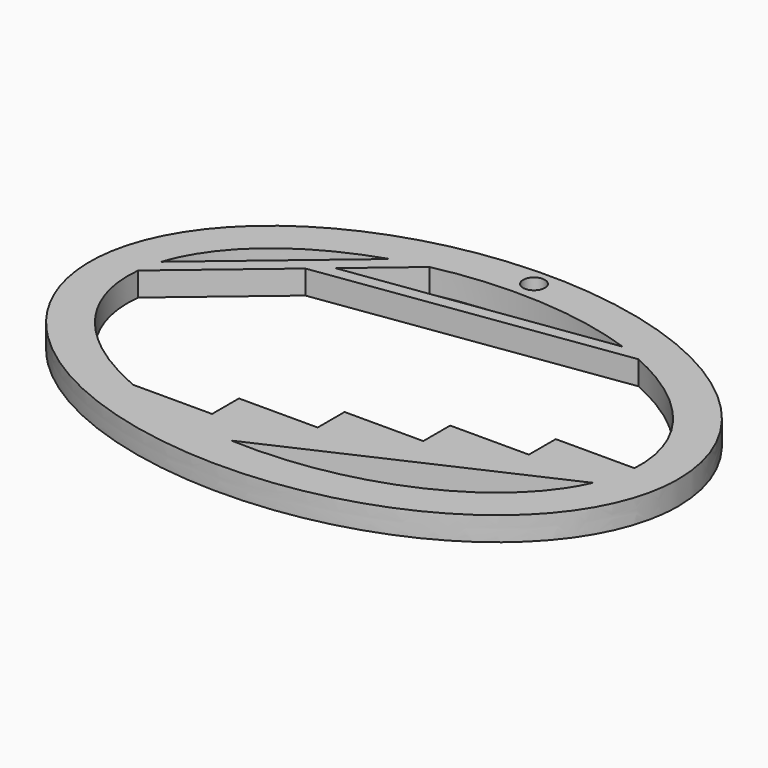
from build123d import *

# Parameters (mm, degrees)
F0_R     = 2.9092310145
F1_DEPTH = 6.35


# Not quite as in the source:
# - the dataset's text gives a spline's control points without its knots; the knots are read off the source's solid


with BuildPart() as f1:
    # F0 (on Top) → F1 (new body)
    with BuildSketch(Plane.XY):
        with BuildLine():
            add(Edge.make_bspline(
                [(35.9756101214, 33.5026877272), (35.9756101214, 34.4984874099), (35.8998248814, 36.4900867753), (35.4503858288, 40.4322788005), (34.3434038279, 45.2628804916), (32.2018791957, 50.8187815017), (29.3153723523, 56.0785646116), (25.7483483064, 61.007460002), (21.5563607444, 65.5851842551), (17.578902898, 69.0969458075), (14.1259575568, 71.7179929744), (11.4002575101, 73.5909345896), (8.5592861675, 75.3582652241), (4.6489563898, 77.560297414), (-0.4640075549, 80.0325432498), (-6.9121068292, 82.5530431102), (-13.6323017507, 84.628618245), (-20.5844989833, 86.2564877673), (-27.7291202294, 87.4311380236), (-33.8116403616, 88.02561485), (-38.7328840311, 88.2654165363), (-42.4521933959, 88.3258891821), (-46.1715027606, 88.2654165363), (-51.0927464301, 88.02561485), (-57.1752665623, 87.4311380236), (-64.3198878084, 86.2564877673), (-71.272085041, 84.628618245), (-77.9922799626, 82.5530431102), (-84.4403792369, 80.0325432498), (-89.5533431816, 77.560297414), (-93.4636729593, 75.3582652241), (-96.3046443018, 73.5909345896), (-99.0303443486, 71.7179929744), (-102.4832896898, 69.0969458075), (-106.4607475362, 65.5851842551), (-110.6527350981, 61.007460002), (-114.219759144, 56.0785646116), (-117.1062659874, 50.8187815017), (-119.2477906196, 45.2628804916), (-120.3547726206, 40.4322788005), (-120.8042116732, 36.4900867753), (-120.917889533, 33.5026877272), (-120.8042116732, 30.5152886791), (-120.3547726206, 26.5730966538), (-119.2477906196, 21.7424949627), (-117.1062659874, 16.1865939527), (-114.219759144, 10.9268108427), (-110.6527350981, 5.9979154523), (-106.4607475362, 1.4201911992), (-102.4832896898, -2.0915703531), (-99.0303443486, -4.7126175201), (-96.3046443018, -6.5855591353), (-93.4636729593, -8.3528897698), (-89.5533431816, -10.5549219597), (-84.4403792369, -13.0271677955), (-77.9922799626, -15.5476676559), (-71.272085041, -17.6232427907), (-64.3198878084, -19.251112313), (-57.1752665623, -20.4257625693), (-51.0927464301, -21.0202393957), (-46.1715027606, -21.260041082), (-42.4521933959, -21.3205137277), (-38.7328840311, -21.260041082), (-33.8116403616, -21.0202393957), (-27.7291202294, -20.4257625693), (-20.5844989833, -19.251112313), (-13.6323017507, -17.6232427907), (-6.9121068292, -15.5476676559), (-0.4640075549, -13.0271677955), (4.6489563898, -10.5549219597), (8.5592861675, -8.3528897698), (11.4002575101, -6.5855591353), (14.1259575568, -4.7126175201), (17.578902898, -2.0915703531), (21.5563607444, 1.4201911992), (25.7483483064, 5.9979154523), (29.3153723523, 10.9268108427), (32.2018791957, 16.1865939527), (34.3434038279, 21.7424949627), (35.4503858288, 26.5730966538), (35.8998248814, 30.5152886791), (35.9756101214, 32.5068880445), (35.9756101214, 33.5026877272)],
                knots=[0, 0, 0, 0, 0.0078125, 0.015625, 0.03125, 0.046875, 0.0625, 0.078125, 0.09375, 0.109375, 0.1171875, 0.125, 0.1328125, 0.140625, 0.15625, 0.171875, 0.1875, 0.203125, 0.21875, 0.234375, 0.2421875, 0.25, 0.2578125, 0.265625, 0.28125, 0.296875, 0.3125, 0.328125, 0.34375, 0.359375, 0.3671875, 0.375, 0.3828125, 0.390625, 0.40625, 0.421875, 0.4375, 0.453125, 0.46875, 0.484375, 0.4921875, 0.5, 0.5078125, 0.515625, 0.53125, 0.546875, 0.5625, 0.578125, 0.59375, 0.609375, 0.6171875, 0.625, 0.6328125, 0.640625, 0.65625, 0.671875, 0.6875, 0.703125, 0.71875, 0.734375, 0.7421875, 0.75, 0.7578125, 0.765625, 0.78125, 0.796875, 0.8125, 0.828125, 0.84375, 0.859375, 0.8671875, 0.875, 0.8828125, 0.890625, 0.90625, 0.921875, 0.9375, 0.953125, 0.96875, 0.984375, 0.9921875, 1, 1, 1, 1], degree=3))
        make_face()
        with BuildLine():
            add(Edge.make_bspline(
                [(25.8156101214, 33.5026877272), (25.8156101214, 57.2508032081), (-4.2990424349, 70.5230250799)],
                knots=[0, 0, 0, 0.9777681056, 0.9777681056, 0.9777681056], degree=2, weights=[1, 0.8828575027, 1]))
            add(Edge.make_bspline(
                [(25.7583993431, 31.6753923662), (25.8156101214, 32.588657052), (25.8156101214, 33.5026877272)],
                knots=[6.2422426246, 6.2422426246, 6.2422426246, 6.2831853072, 6.2831853072, 6.2831853072], degree=2, weights=[1, 0.9997904694, 1]))
            add(Edge.make_bspline(
                [(23.1351877715, 21.1159459884), (25.4211705669, 26.2921561677), (25.7583993431, 31.6753923662)],
                knots=[6.0020340843, 6.0020340843, 6.0020340843, 6.2422426246, 6.2422426246, 6.2422426246], degree=2, weights=[1, 0.9927961481, 1]))
            add(Edge.make_bspline(
                [(-47.5005840408, -11.0181219568), (7.7603026977, -13.6978053575), (23.1351877715, 21.1159459884)],
                knots=[4.6383716106, 4.6383716106, 4.6383716106, 6.0020340843, 6.0020340843, 6.0020340843], degree=2, weights=[1, 0.7764199467, 1]))
            add(Edge.make_bspline(
                [(-79.1219276756, -4.1532595133), (-64.6320440132, -10.187391731), (-47.5005840408, -11.0181219568)],
                knots=[4.1453398468, 4.1453398468, 4.1453398468, 4.6383716106, 4.6383716106, 4.6383716106], degree=2, weights=[1, 0.9697685237, 1]))
            add(Edge.make_bspline(
                [(-110.5443222079, 36.703320692), (-113.4632203195, 10.1477455995), (-79.1219276756, -4.1532595133)],
                knots=[3.0698372147, 3.0698372147, 3.0698372147, 4.1453398468, 4.1453398468, 4.1453398468], degree=2, weights=[1, 0.8588626412, 1]))
            add(Edge.make_bspline(
                [(-109.2216839605, 42.8044663438), (-110.2057251662, 39.7838116244), (-110.5443222079, 36.703320692)],
                knots=[2.9316958501, 2.9316958501, 2.9316958501, 3.0698372147, 3.0698372147, 3.0698372147], degree=2, weights=[1, 0.9976155686, 1]))
            add(Edge.make_bspline(
                [(-72.8862277584, 73.4640507782), (-102.3608878748, 63.8646576809), (-109.2216839605, 42.8044663438)],
                knots=[2.0328681623, 2.0328681623, 2.0328681623, 2.9316958501, 2.9316958501, 2.9316958501], degree=2, weights=[1, 0.9007019054, 1]))
            add(Edge.make_bspline(
                [(-64.1814982473, 75.8239225616), (-68.6586891877, 74.8408878448), (-72.8862277584, 73.4640507782)],
                knots=[1.8947267977, 1.8947267977, 1.8947267977, 2.0328681623, 2.0328681623, 2.0328681623], degree=2, weights=[1, 0.9976155686, 1]))
            add(Edge.make_bspline(
                [(-10.329989388, 72.8949414232), (-36.2906029544, 81.9477887805), (-64.1814982473, 75.8239225616)],
                knots=[1.0809024359, 1.0809024359, 1.0809024359, 1.8947267977, 1.8947267977, 1.8947267977], degree=2, weights=[1, 0.9183472822, 1]))
            add(Edge.make_bspline(
                [(-4.2990424349, 70.5230250799), (-7.2209128714, 71.8107607641), (-10.329989388, 72.8949414232)],
                knots=[0.9777681056, 0.9777681056, 0.9777681056, 1.0809024359, 1.0809024359, 1.0809024359], degree=2, weights=[1, 0.9986707083, 1]))
        make_face(mode=Mode.SUBTRACT)
        with Locations((-42.4521933959, 83.4672963517)):
            Circle(F0_R, mode=Mode.SUBTRACT)
        with BuildLine():
            Line((-110.5443222079, 36.703320692), (-83.941566481, 59.1505257266))
            Line((-83.941566481, 59.1505257266), (-79.1567558079, 63.1879129557))
            Line((-79.1567558079, 63.1879129557), (-64.1814982473, 75.8239225616))
            add(Edge.make_bspline(
                [(-64.1814982473, 75.8239225616), (-68.6586891877, 74.8408878448), (-72.8862277584, 73.4640507782)],
                knots=[1.8947267977, 1.8947267977, 1.8947267977, 2.0328681623, 2.0328681623, 2.0328681623], degree=2, weights=[1, 0.9976155686, 1]))
            Line((-72.8862277584, 73.4640507782), (-109.2216839605, 42.8044663438))
            add(Edge.make_bspline(
                [(-109.2216839605, 42.8044663438), (-110.2057251662, 39.7838116244), (-110.5443222079, 36.703320692)],
                knots=[2.9316958501, 2.9316958501, 2.9316958501, 3.0698372147, 3.0698372147, 3.0698372147], degree=2, weights=[1, 0.9976155686, 1]))
        make_face()
        with BuildLine():
            Line((-83.941566481, 59.1505257266), (-4.2990424349, 70.5230250799))
            add(Edge.make_bspline(
                [(-4.2990424349, 70.5230250799), (-7.2209128714, 71.8107607641), (-10.329989388, 72.8949414232)],
                knots=[0.9777681056, 0.9777681056, 0.9777681056, 1.0809024359, 1.0809024359, 1.0809024359], degree=2, weights=[1, 0.9986707083, 1]))
            Line((-10.329989388, 72.8949414232), (-79.1567558079, 63.1879129557))
            Line((-79.1567558079, 63.1879129557), (-83.941566481, 59.1505257266))
        make_face()
        with BuildLine():
            add(Edge.make_bspline(
                [(23.1351877715, 21.1159459884), (25.4211705669, 26.2921561677), (25.7583993431, 31.6753923662)],
                knots=[6.0020340843, 6.0020340843, 6.0020340843, 6.2422426246, 6.2422426246, 6.2422426246], degree=2, weights=[1, 0.9927961481, 1]))
            Line((25.7583993431, 31.6753923662), (6.8798116408, 31.6753923662))
            Line((6.8798116408, 31.6753923662), (5.5530862883, 31.6753923662))
            Line((5.5530862883, 31.6753923662), (4.7823339394, 31.6753923662))
            Line((4.7823339394, 31.6753923662), (4.7823339394, 22.7182293963))
            Line((4.7823339394, 22.7182293963), (-16.1937314644, 22.7182293963))
            Line((-16.1937314644, 22.7182293963), (-16.1937314644, 13.7610664264))
            Line((-16.1937314644, 13.7610664264), (-37.1697968681, 13.7610664264))
            Line((-37.1697968681, 13.7610664264), (-37.1697968681, 4.8039034566))
            Line((-37.1697968681, 4.8039034566), (-58.1458622718, 4.8039034566))
            Line((-58.1458622718, 4.8039034566), (-58.1458622718, -4.1532595133))
            Line((-58.1458622718, -4.1532595133), (-79.1219276756, -4.1532595133))
            add(Edge.make_bspline(
                [(-79.1219276756, -4.1532595133), (-64.6320440132, -10.187391731), (-47.5005840408, -11.0181219568)],
                knots=[4.1453398468, 4.1453398468, 4.1453398468, 4.6383716106, 4.6383716106, 4.6383716106], degree=2, weights=[1, 0.9697685237, 1]))
            Line((-47.5005840408, -11.0181219568), (23.1351877715, 21.1159459884))
        make_face()
    extrude(amount=-F1_DEPTH)


solid = f1.part
